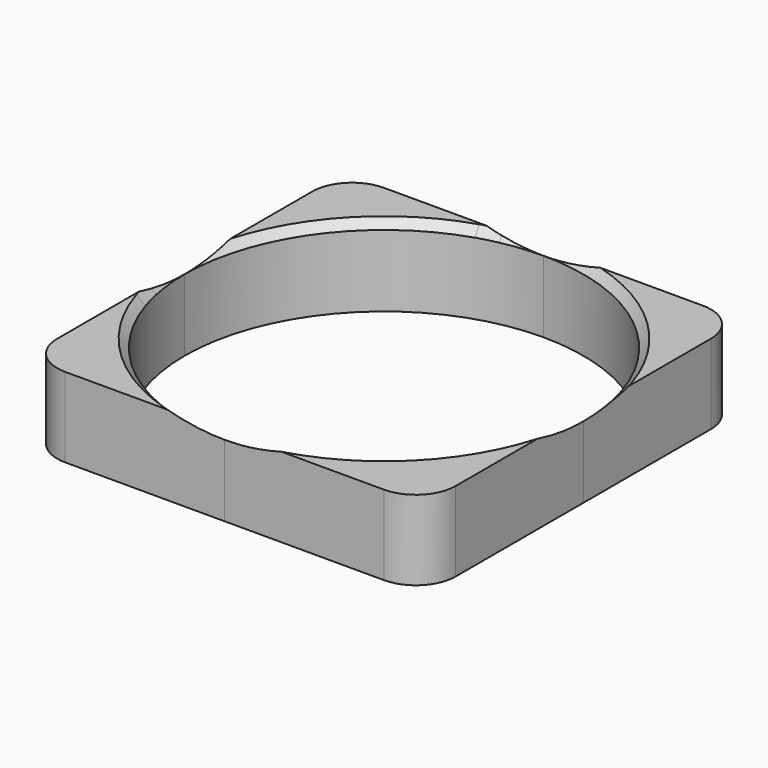
from build123d import *

# Parameters (mm, degrees)
F0_W           = 50
F0_H           = 50
F1_DEPTH       = 10
F3_DEPTH       = 10.001
F4_R           = 5
F5_T2_ANGLE    = 125.3773855197
F5_S1_T2_ANGLE = 95.892873339
F5_S2_T2_ANGLE = 95.8953917499
F5_S3_T2_ANGLE = 66.4146031024


# Not quite as in the source:
# - a fillet or chamfer that OpenCascade refuses, or shapes differently, is made with other operations: its cross-section is extruded or revolved along the edge and cut away or added


with BuildPart() as f1:
    # F0 (on Top) → F1 (new body)
    with BuildSketch(Plane.XY):
        Rectangle(F0_W, F0_H)
    extrude(amount=F1_DEPTH)

    # F2 (on face) → F3 (cut, through all)
    with BuildSketch(Plane.XY.offset(10)):
        with BuildLine():
            ThreePointArc((-5.83e-08, -25), (17.677669509, -17.6776695503), (25, 0))
            ThreePointArc((25, 0), (17.6776695297, 17.6776695297), (0, 25))
            ThreePointArc((0, 25), (-17.6776695204, 17.6776695389), (-25, 2.61e-08))
            ThreePointArc((-25, 2.61e-08), (-17.6776695595, -17.6776694998), (-5.83e-08, -25))
        make_face()
    extrude(amount=-F3_DEPTH, mode=Mode.SUBTRACT)

    # F4
    f4_edges = [f1.edges().sort_by_distance(p)[0] for p in [
        (25, -25, 5),
        (25, 25, 5),
        (-25, 25, 5),
        (-25, -25, 5),
    ]]
    fillet(f4_edges, radius=F4_R)

    # F5: chamfer of 1 on 1 edges, made by hand

    # F5_s1 → F5_t2 (revolve, cut)
    with BuildSketch(Plane(origin=(0, 0, 0), x_dir=(0, 0, 1), z_dir=(-0.3038450488, 0.9527214631, 0))):
        Polygon((9, 25), (10, 26), (10, 25), align=None)
    revolve(axis=Axis((0, 0, 10), (0, 0, -1)), revolution_arc=F5_T2_ANGLE, mode=Mode.SUBTRACT)

    # F5#s1: chamfer of 1 on 1 edges, made by hand

    # F5_s1_s1 → F5_s1_t2 (revolve, cut)
    with BuildSketch(Plane(origin=(0, 0, 0), x_dir=(0, 0, 1), z_dir=(-0.9527348163, -0.3038031761, 0))):
        Polygon((10, 26), (9, 25), (10, 25), align=None)
    revolve(axis=Axis((0, 0, 10), (0, 0, -1)), revolution_arc=F5_S1_T2_ANGLE, mode=Mode.SUBTRACT)

    # F5#s2: chamfer of 1 on 1 edges, made by hand

    # F5_s2_s1 → F5_s2_t2 (revolve, cut)
    with BuildSketch(Plane(origin=(0, 0, 0), x_dir=(0, 0, 1), z_dir=(0.3038031783, -0.9527348156, 0))):
        Polygon((10, 26), (9, 25), (10, 25), align=None)
    revolve(axis=Axis((0, 0, 10), (0, 0, -1)), revolution_arc=F5_S2_T2_ANGLE, mode=Mode.SUBTRACT)

    # F5#s3: chamfer of 1 on 1 edges, made by hand

    # F5_s3_s1 → F5_s3_t2 (revolve, cut)
    with BuildSketch(Plane(origin=(0, 0, 0), x_dir=(0, 0, 1), z_dir=(0.9788889499, -0.2043928171, 0))):
        Polygon((10, 26), (9, 25), (10, 25), align=None)
    revolve(axis=Axis((0, 0, 10), (0, 0, -1)), revolution_arc=F5_S3_T2_ANGLE, mode=Mode.SUBTRACT)


solid = f1.part
